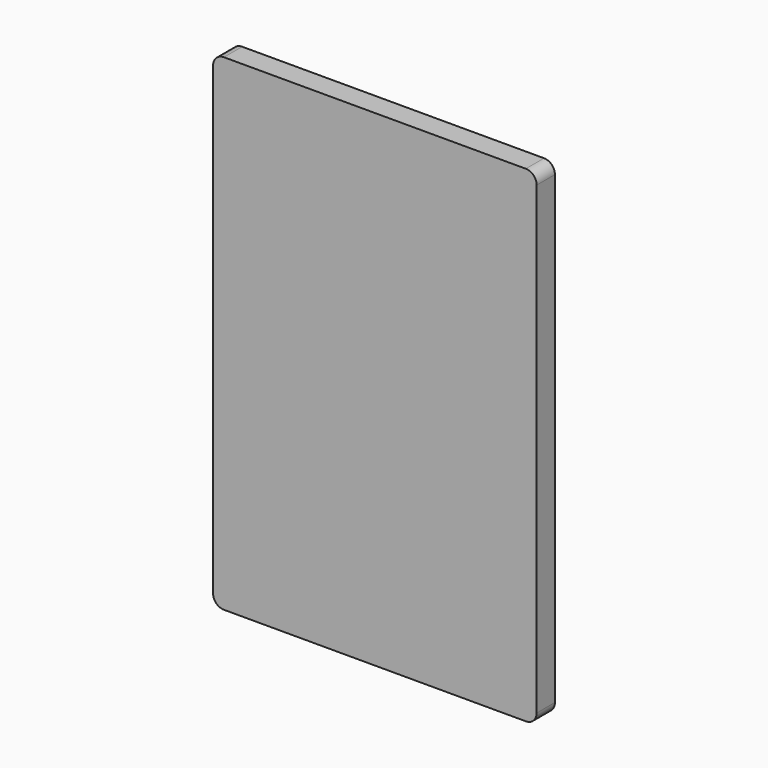
from build123d import *

# Parameters (mm, degrees)
F0_W     = 38
F0_H     = 51
F1_DEPTH = 21
F2_DEPTH = 18
F3_T     = 10


# Not quite as in the source:
# - a shell that OpenCascade refuses in one call is made with other operations: the cavity is built on its own and cut out


with BuildPart() as f1:
    # F0 (on Front) → F1 (new body)
    with BuildSketch(Plane.XZ):
        with BuildLine():
            Line((139, 224), (-139, 224))
            ThreePointArc((-139, 224), (-146.0710678119, 221.0710678119), (-149, 214))
            Line((-149, 214), (-149, -214))
            ThreePointArc((-149, -214), (-146.0710678119, -221.0710678119), (-139, -224))
            Line((-139, -224), (139, -224))
            ThreePointArc((139, -224), (146.0710678119, -221.0710678119), (149, -214))
            Line((149, -214), (149, 214))
            ThreePointArc((149, 214), (146.0710678119, 221.0710678119), (139, 224))
        make_face()
        with Locations((0, -188.5)):
            Rectangle(F0_W, F0_H, mode=Mode.SUBTRACT)
        with Locations((0, -188.5)):
            Rectangle(F0_W, F0_H)
    extrude(amount=F1_DEPTH)

    # F3: shell of thickness 10, made by hand


with BuildPart() as f2:
    # F0 (on Front) → F2 (new body)
    with BuildSketch(Plane.XZ):
        with Locations((0, -188.5)):
            Rectangle(F0_W, F0_H)
    extrude(amount=F2_DEPTH)


with BuildPart() as f3_core1:
    # F3_t2: copy of F1
    add(f1.part)

    # the walls: a layer under each face that stays
    f3_faces = [f3_core1.faces().sort_by_distance(p)[0] for p in [
        (0, -10.5, 224),
        (-149, -10.5, 0),
        (0, -10.5, -224),
        (149, -10.5, 0),
        (0, -21, 0),
    ]]
    thicken(f3_faces, amount=-F3_T, mode=Mode.SUBTRACT)


with BuildPart() as f1_1:
    add(f1.part)

    # what is left inside the walls is the cavity
    f3_cavity = [f3_core1.part.solids().sort_by_distance(p)[0] for p in [
        (0, -0.1, -71.333333),
    ]]
    add(f3_cavity, mode=Mode.SUBTRACT)


solid = Compound([f2.part, f1_1.part])
